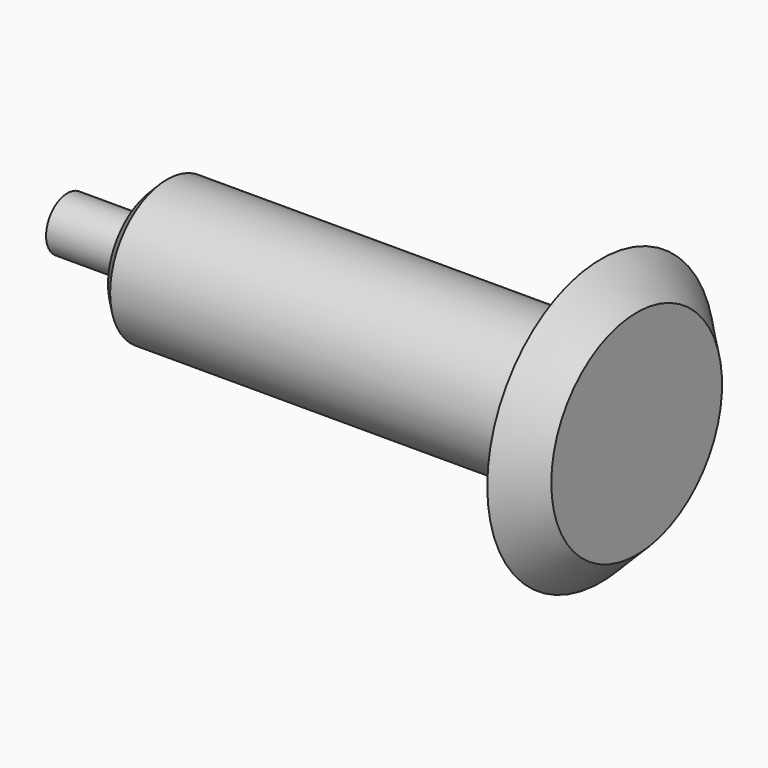
from build123d import *

# Parameters (mm, degrees)
F2_SIZE2 = 3
F2_SIZE  = 3
F3_SIZE2 = 10
F3_SIZE  = 10
F4_SIZE2 = 9.99999
F4_SIZE  = 9.99999


# Not quite as in the source:
# - a fillet or chamfer is up to 0.001 mm smaller than in the source, because OpenCascade refuses the exact size


with BuildPart() as f1:
    # F0 (on Top) → F1 (revolve)
    with BuildSketch(Plane.XY):
        Polygon((160, 0), (0, 0), (0, -7.5), (25, -7.5), (25, -20), (150, -20), (150, -40), (160, -40), align=None)
    revolve(axis=Axis((80, 0, 0), (-1, 0, 0)))

    # F2
    f2_edges = [f1.edges().sort_by_distance(p)[0] for p in [
        (25, 20, 0),
    ]]
    chamfer(f2_edges, length=F2_SIZE, length2=F2_SIZE2)

    # F3
    f3_edges = [f1.edges().sort_by_distance(p)[0] for p in [
        (150, 20, 0),
    ]]
    chamfer(f3_edges, length=F3_SIZE, length2=F3_SIZE2)

    # F4 (size 10 and 10 in the source; OpenCascade refuses exactly that, so slightly less here)
    f4_edges = [f1.edges().sort_by_distance(p)[0] for p in [
        (160, 40, 0),
    ]]
    chamfer(f4_edges, length=F4_SIZE, length2=F4_SIZE2)


solid = f1.part
